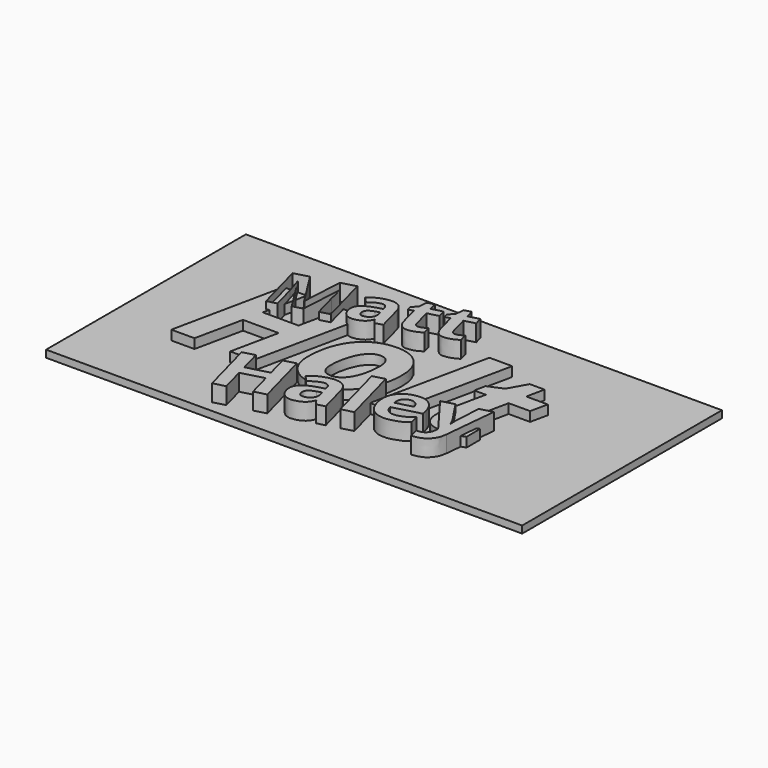
from build123d import *

# Parameters (mm, degrees)
F0_TEXT_SIZE = 82.7294256952
F3_DEPTH     = 8.89
F1_TEXT_SIZE = 38.4978536103
F4_DEPTH     = 12.7
F2_TEXT_SIZE = 42.866398063
F5_DEPTH     = 12.7
F6_W         = 253.4110993147
F6_H         = 132.9021565616
F7_DEPTH     = 3.81


# Not quite as in the source:
# - Text() gives the source's letters only with a copy of the font that has no kerning and outlines rounded to 1/6400 em; it was checked with that copy


with BuildPart() as f3:
    # F0 (on Top) → F3 (new body)
    with BuildSketch(Plane.XY):
        with Locations((-87.1135666966, -31.5756071359)):
            Text('Holt', F0_TEXT_SIZE, font='Open Sans', font_style=FontStyle.BOLDITALIC, text_align=(TextAlign.LEFT, TextAlign.BOTTOM))
    extrude(amount=F3_DEPTH)


with BuildPart() as f4:
    # F1 (on Top) → F4 (new body)
    with BuildSketch(Plane.XY):
        with Locations(Location((-69.04191036, 6.4772344891), (0, 0, 15))):
            Text('Matt', F1_TEXT_SIZE, font='Open Sans', font_style=FontStyle.BOLD, text_align=(TextAlign.LEFT, TextAlign.BOTTOM))
    extrude(amount=F4_DEPTH)


with BuildPart() as f5:
    # F2 (on Top) → F5 (new body)
    with BuildSketch(Plane.XY):
        with Locations(Location((-40.7498090905, -65.4229252295), (0, 0, 15))):
            Text('Haley', F2_TEXT_SIZE, font='Open Sans', font_style=FontStyle.BOLD, text_align=(TextAlign.LEFT, TextAlign.BOTTOM))
    extrude(amount=F5_DEPTH)


with BuildPart() as f7:
    # F6 (on Top) → F7 (new body)
    with BuildSketch(Plane.XY):
        with Locations((6.2365308404, -4.0811914951)):
            Rectangle(F6_W, F6_H)
    extrude(amount=F7_DEPTH)


solid = Compound([f3.part, f4.part, f5.part, f7.part])
